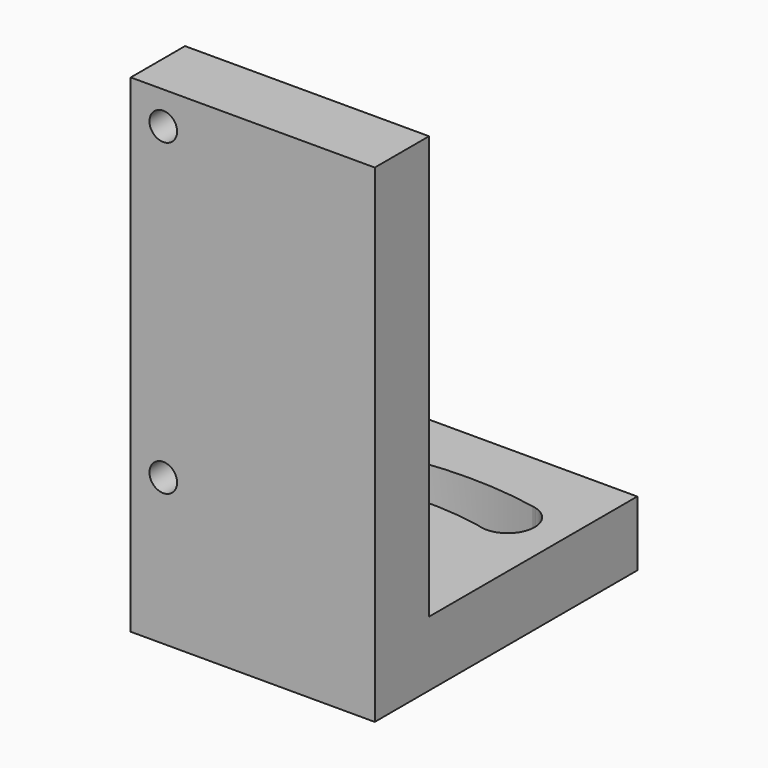
from build123d import *

# Parameters (mm, degrees)
F1_DEPTH = 30
F3_D     = 3.4
F5_DEPTH = 25
F6_D     = 6.6


# Not quite as in the source:
# - a feature names something its author has since deleted; it is built from what else it names


with BuildPart() as f1:
    # F0 (on Right) → F1 (new body)
    with BuildSketch(Plane.YZ):
        Polygon((0, 60), (0, 0), (40.3389412612, 0), (40.3389412612, 8), (8.3389412612, 8), (8.3389412612, 60), align=None)
    extrude(amount=F1_DEPTH)

    # F3 (through all)
    with Locations(Plane.XZ):
        with Locations((4, 56), (4, 18)):
            Hole(F3_D / 2)

    # F4 (on face) → F5 (cut)
    with BuildSketch(Plane(origin=(0, 0, 0), x_dir=(1, 0, 0), z_dir=(0, 0, -1))):
        with BuildLine():
            ThreePointArc((8.2706560702, -26.1462763052), (7.66, -25.9585094241), (7.0246071276, -25.8919276299))
            ThreePointArc((7.0246071276, -25.8919276299), (7.6465318102, -26.0244898096), (8.2706560702, -26.1462763052))
        make_face()
        with BuildLine():
            ThreePointArc((22.9753928724, -25.8919276299), (22.34, -25.9585094241), (21.7293439298, -26.1462763052))
            ThreePointArc((21.7293439298, -26.1462763052), (22.3534681898, -26.0244898096), (22.9753928724, -25.8919276299))
        make_face()
        with BuildLine():
            ThreePointArc((19.7422005642, -29.7178994133), (15, -30), (10.2577994358, -29.7178994133))
            ThreePointArc((10.2577994358, -29.7178994133), (8.9379952514, -31.8628234183), (6.4894588415, -32.4521039296))
            ThreePointArc((6.4894588415, -32.4521039296), (15, -33.2967716909), (23.5105411585, -32.4521039296))
            ThreePointArc((23.5105411585, -32.4521039296), (21.0620047486, -31.8628234183), (19.7422005642, -29.7178994133))
        make_face()
        with BuildLine():
            ThreePointArc((10.3, -29.1918358845), (10.2894329403, -29.455712619), (10.2577994358, -29.7178994133))
            ThreePointArc((10.2577994358, -29.7178994133), (15, -30), (19.7422005642, -29.7178994133))
            ThreePointArc((19.7422005642, -29.7178994133), (20.1162784073, -27.5874201728), (21.7293439298, -26.1462763052))
            ThreePointArc((21.7293439298, -26.1462763052), (15, -26.767340949), (8.2706560702, -26.1462763052))
            ThreePointArc((8.2706560702, -26.1462763052), (9.7461941876, -27.3619677242), (10.3, -29.1918358845))
        make_face()
        with BuildLine():
            ThreePointArc((7.0246071276, -25.8919276299), (4.9757761074, -26.5855899958), (3.7966505642, -28.3990229227))
            ThreePointArc((3.7966505642, -28.3990229227), (7, -29.1918358845), (10.2577994358, -29.7178994133))
            ThreePointArc((10.2577994358, -29.7178994133), (10.2894329403, -29.455712619), (10.3, -29.1918358845))
            ThreePointArc((10.3, -29.1918358845), (9.7461941876, -27.3619677242), (8.2706560702, -26.1462763052))
            ThreePointArc((8.2706560702, -26.1462763052), (7.6465318102, -26.0244898096), (7.0246071276, -25.8919276299))
        make_face()
        with BuildLine():
            ThreePointArc((10.2577994358, -29.7178994133), (7, -29.1918358845), (3.7966505642, -28.3990229227))
            ThreePointArc((3.7966505642, -28.3990229227), (4.170235318, -30.8896084972), (6.1919389643, -32.3913729389))
            ThreePointArc((6.1919389643, -32.3913729389), (6.3406456618, -32.421999261), (6.4894588415, -32.4521039296))
            ThreePointArc((6.4894588415, -32.4521039296), (8.9379952514, -31.8628234183), (10.2577994358, -29.7178994133))
        make_face()
        with BuildLine():
            ThreePointArc((26.2033494358, -28.3990229227), (23, -29.1918358845), (19.7422005642, -29.7178994133))
            ThreePointArc((19.7422005642, -29.7178994133), (21.0620047486, -31.8628234183), (23.5105411585, -32.4521039296))
            ThreePointArc((23.5105411585, -32.4521039296), (23.6593543382, -32.421999261), (23.8080610357, -32.3913729389))
            ThreePointArc((23.8080610357, -32.3913729389), (25.6035169884, -31.2195684337), (26.3, -29.1918358845))
            ThreePointArc((26.3, -29.1918358845), (26.2757482457, -28.7924946382), (26.2033494358, -28.3990229227))
        make_face()
        with BuildLine():
            ThreePointArc((21.7293439298, -26.1462763052), (20.1162784073, -27.5874201728), (19.7422005642, -29.7178994133))
            ThreePointArc((19.7422005642, -29.7178994133), (23, -29.1918358845), (26.2033494358, -28.3990229227))
            ThreePointArc((26.2033494358, -28.3990229227), (25.0242238926, -26.5855899958), (22.9753928724, -25.8919276299))
            ThreePointArc((22.9753928724, -25.8919276299), (22.3534681898, -26.0244898096), (21.7293439298, -26.1462763052))
        make_face()
    extrude(amount=-F5_DEPTH, mode=Mode.SUBTRACT)

    # F6 (through all)
    with Locations(Plane(origin=(0, 0, 0), x_dir=(1, 0, 0), z_dir=(0, 0, -1))):
        with Locations((15, -15)):
            Hole(F6_D / 2)


solid = f1.part
